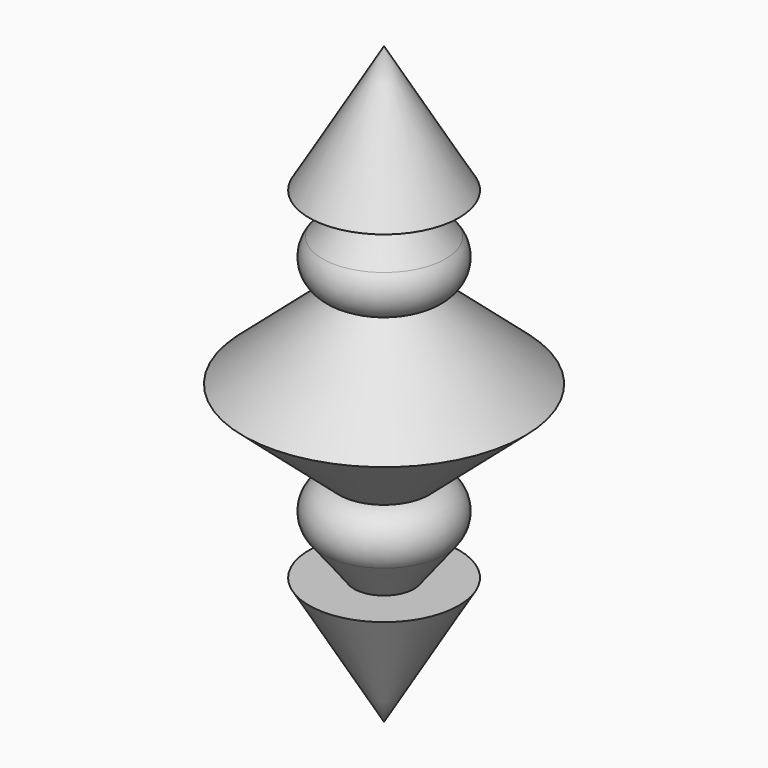
from build123d import *


# Not quite as in the source:
# - a fillet or chamfer that OpenCascade refuses, or shapes differently, is made with other operations: its cross-section is extruded or revolved along the edge and cut away or added


with BuildPart() as f1:
    # F0 (on Front) → F1 (revolve)
    with BuildSketch(Plane.XZ):
        Polygon((12.6077588648, 28.7068989128), (0, 50.0431060791), (0, -9.1163795441), (3.6853442434, -9.1163795441), (3.6853442434, 0), (23.6637946218, 0), (7.5646545738, 13.9655172825), (16.487069428, 13.9655172825), (5.043104291, 28.7068989128), align=None)
    revolve(axis=Axis((0, 0, 20.4633632675), (0, 0, 1)))


with BuildPart() as f2_1:
    # F2: instance of F1
    add(f1.part.mirror(Plane.XY))

    # F4: fillet of radius 5 on 1 edges, made by hand

    # F4_s1 → F4_t2 (revolve, cut)
    with BuildSketch(Plane.XZ):
        with BuildLine():
            ThreePointArc((7.5646545738, -13.9655172825), (11.1051748853, -17.1745962427), (10.3347655016, -21.8905204608))
            Line((10.3347655016, -21.8905204608), (16.487069428, -13.9655172825))
            Line((16.487069428, -13.9655172825), (7.5646545738, -13.9655172825))
        make_face()
    revolve(axis=Axis((0, 0, -13.9655172825), (0, 0, 1)), mode=Mode.SUBTRACT)


with BuildPart() as f1_1:
    add(f1.part)

    # F3: fillet of radius 5 on 1 edges, made by hand

    # F3_s1 → F3_t2 (revolve, cut)
    with BuildSketch(Plane.XZ):
        with BuildLine():
            ThreePointArc((7.5646545738, 13.9655172825), (11.1051748853, 17.1745962427), (10.3347655016, 21.8905204608))
            Line((10.3347655016, 21.8905204608), (16.487069428, 13.9655172825))
            Line((16.487069428, 13.9655172825), (7.5646545738, 13.9655172825))
        make_face()
    revolve(axis=Axis((0, 0, 13.9655172825), (0, 0, 1)), mode=Mode.SUBTRACT)


solid = Compound([f2_1.part, f1_1.part])
